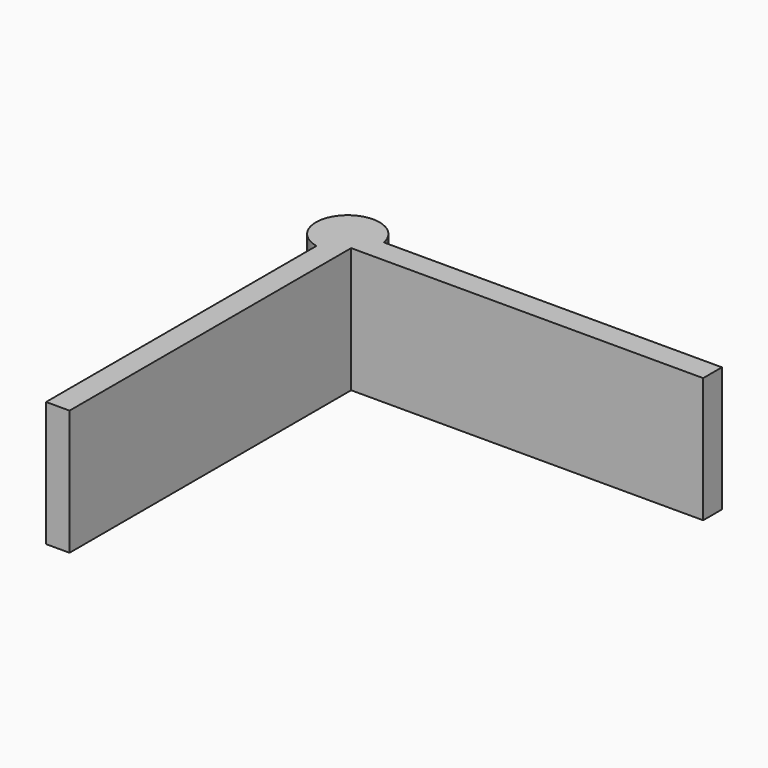
from build123d import *

# Parameters (mm, degrees)
F1_DEPTH = 25.4


# Not quite as in the source:
# - a feature names something its author has since deleted; it is built from what else it names


with BuildPart() as f1:
    # F0 (on Top) → F1 (new body)
    with BuildSketch(Plane.XY):
        Polygon((-32.0039994973, 49.1343741807), (-39.6239994973, 49.1343741807), (-39.6239994973, 41.5143741807), (-39.6239994973, -27.0656258193), (-34.8614994973, -27.0656258193), (-34.8614994973, 44.3718741807), (36.5760005027, 44.3718741807), (36.5760005027, 49.1343741807), align=None)
        with BuildLine():
            Line((-39.6239994973, 41.5143741807), (-39.6239994973, 49.1343741807))
            Line((-39.6239994973, 49.1343741807), (-32.0039994973, 49.1343741807))
            ThreePointArc((-32.0039994973, 49.1343741807), (-42.8727293035, 52.3831039869), (-39.6239994973, 41.5143741807))
        make_face()
    extrude(amount=F1_DEPTH)


solid = f1.part
